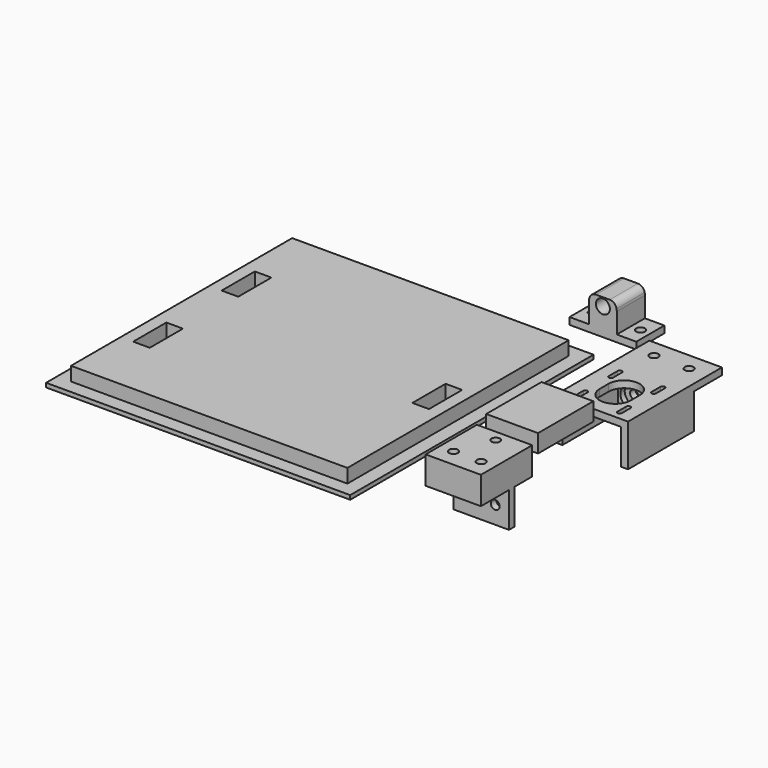
from build123d import *

# Parameters (mm, degrees)
F2_R      = 5.05
F3_DEPTH  = 25.4
F4_R      = 3.2
F5_DEPTH  = 5
F6_W      = 42.5
F6_H      = 50.5
F6_W_2    = 52.5
F6_H_2    = 25.4
F6_R      = 3.2
F7_DEPTH  = 5
F8_DEPTH  = 25.4
F9_R      = 3.2
F10_DEPTH = 9
F9_R_2    = 7.05
F11_DEPTH = 4
F12_W     = 40
F12_H     = 25.4
F12_R     = 3.2
F13_DEPTH = 15
F12_R_2   = 3.05
F14_DEPTH = 5
F15_R     = 3.2
F15_R_2   = 3.05
F16_DEPTH = 5
F17_DEPTH = 25.4
F18_R     = 3.2
F19_DEPTH = 5
F20_R     = 5.05
F20_R_2   = 3.05
F22_DEPTH = 1
F21_R     = 5.05
F21_R_2   = 3.05
F23_DEPTH = 1
F24_SIZE  = 0.99999
F26_W     = 18.7451829227
F26_H     = 8
F27_DEPTH = 25
F29_DEPTH = 8
F30_W     = 220
F30_H     = 220
F30_W_2   = 12
F30_H_2   = 30
F31_DEPTH = 3
F34_W     = 200
F34_H     = 200
F34_W_2   = 12
F34_H_2   = 30
F35_DEPTH = 10


# Not quite as in the source:
# - a fillet or chamfer is up to 0.001 mm smaller than in the source, because OpenCascade refuses the exact size
# - a feature names something its author has since deleted; it is built from what else it names


with BuildPart() as f3:
    # F2 (on offset) → F3 (new body)
    with BuildSketch(Plane.XZ.offset(-50)):
        Polygon((-65.3854490548, 5), (-79.4854490548, 5), (-79.4854490548, 0), (-31.1854490548, 0), (-31.1854490548, 5), (-45.2854490548, 5), align=None)
        with BuildLine():
            Line((-65.3854490548, 19.6345400687), (-65.3854490548, 5))
            Line((-65.3854490548, 5), (-45.2854490548, 5))
            Line((-45.2854490548, 5), (-45.2854490548, 19.6345400687))
            ThreePointArc((-45.2854490548, 19.6345400687), (-55.3354490548, 9.5845400687), (-65.3854490548, 19.6345400687))
        make_face()
        with BuildLine():
            ThreePointArc((-65.2367624625, 21.3568910211), (-65.3482084085, 20.4989185312), (-65.3854490548, 19.6345400687))
            ThreePointArc((-65.3854490548, 19.6345400687), (-55.3354490548, 9.5845400687), (-45.2854490548, 19.6345400687))
            ThreePointArc((-45.2854490548, 19.6345400687), (-45.3226897012, 20.4989185312), (-45.4341356472, 21.3568910211))
            ThreePointArc((-45.4341356472, 21.3568910211), (-47.1418128824, 24.326516373), (-50.3601622182, 25.5))
            Line((-50.3601622182, 25.5), (-60.3107358915, 25.5))
            ThreePointArc((-60.3107358915, 25.5), (-63.5290852273, 24.326516373), (-65.2367624625, 21.3568910211))
        make_face()
        with Locations((-55.3354490548, 19.6345400687)):
            Circle(F2_R, mode=Mode.SUBTRACT)
    extrude(amount=-F3_DEPTH)

    # F4 (on face) → F5 (cut, through all)
    with BuildSketch(Plane.XY.offset(5)):
        with Locations((-72.4354490548, 62.7)):
            Circle(F4_R)
        with Locations((-38.2354490548, 62.7)):
            Circle(F4_R)
    extrude(amount=-F5_DEPTH, mode=Mode.SUBTRACT)


with BuildPart() as f7:
    # F6 (on Top) → F7 (new body)
    with BuildSketch(Plane.XY):
        with Locations((0, -4)):
            Rectangle(F6_W, F6_H)
        with BuildLine():
            Line((-17.05, -23.5), (-17.05, -15.5))
            ThreePointArc((-17.05, -15.5), (-15.5, -13.95), (-13.95, -15.5))
            Line((-13.95, -15.5), (-13.95, -23.5))
            ThreePointArc((-13.95, -23.5), (-15.5, -25.05), (-17.05, -23.5))
        make_face(mode=Mode.SUBTRACT)
        with BuildLine():
            Line((-17.05, 7.5), (-17.05, 15.5))
            ThreePointArc((-17.05, 15.5), (-15.5, 17.05), (-13.95, 15.5))
            Line((-13.95, 15.5), (-13.95, 7.5))
            ThreePointArc((-13.95, 7.5), (-15.5, 5.95), (-17.05, 7.5))
        make_face(mode=Mode.SUBTRACT)
        with BuildLine():
            Line((13.95, -23.5), (13.95, -15.5))
            ThreePointArc((13.95, -15.5), (15.5, -13.95), (17.05, -15.5))
            Line((17.05, -15.5), (17.05, -23.5))
            ThreePointArc((17.05, -23.5), (15.5, -25.05), (13.95, -23.5))
        make_face(mode=Mode.SUBTRACT)
        with BuildLine():
            Line((-11.25, -8), (-11.25, 0))
            ThreePointArc((-11.25, 0), (0, 11.25), (11.25, 0))
            Line((11.25, 0), (11.25, -8))
            ThreePointArc((11.25, -8), (0, -19.25), (-11.25, -8))
        make_face(mode=Mode.SUBTRACT)
        with BuildLine():
            Line((13.95, 7.5), (13.95, 15.5))
            ThreePointArc((13.95, 15.5), (15.5, 17.05), (17.05, 15.5))
            Line((17.05, 15.5), (17.05, 7.5))
            ThreePointArc((17.05, 7.5), (15.5, 5.95), (13.95, 7.5))
        make_face(mode=Mode.SUBTRACT)
        Polygon((-21.25, 21.25), (21.25, 21.25), (21.25, -29.25), (26.25, -29.25), (26.25, 30.25), (-26.25, 30.25), (-26.25, -29.25), (-21.25, -29.25), align=None)
        with Locations((0, 42.95)):
            Rectangle(F6_W_2, F6_H_2)
        with Locations((-12.7, 42.95)):
            Circle(F6_R, mode=Mode.SUBTRACT)
        with Locations((12.7, 42.95)):
            Circle(F6_R, mode=Mode.SUBTRACT)
    extrude(amount=F7_DEPTH)

    # F6 (on Top) → F8 (join)
    with BuildSketch(Plane.XY):
        Polygon((-21.25, 21.25), (21.25, 21.25), (21.25, -29.25), (26.25, -29.25), (26.25, 30.25), (-26.25, 30.25), (-26.25, -29.25), (-21.25, -29.25), align=None)
    extrude(amount=-F8_DEPTH)

    # F9 (on face) → F10 (cut, through all)
    with BuildSketch(Plane.XZ.offset(-21.25)):
        with Locations((-12.7, -12.7)):
            Circle(F9_R)
        with Locations((12.7, -12.7)):
            Circle(F9_R)
    extrude(amount=-F10_DEPTH, mode=Mode.SUBTRACT)

    # F9 (on face) → F11 (cut)
    with BuildSketch(Plane.XZ.offset(-21.25)):
        with Locations((-12.7, -12.7)):
            Circle(F9_R_2)
        with Locations((-12.7, -12.7)):
            Circle(F9_R, mode=Mode.SUBTRACT)
        with Locations((12.7, -12.7)):
            Circle(F9_R_2)
        with Locations((12.7, -12.7)):
            Circle(F9_R, mode=Mode.SUBTRACT)
    extrude(amount=-F11_DEPTH, mode=Mode.SUBTRACT)


with BuildPart() as f13:
    # F12 (on Top) → F13 (new body)
    with BuildSketch(Plane.XY):
        Polygon((-3.313708499, -124.0808303208), (-20, -124.0808303208), (-20, -129.0808303208), (20, -129.0808303208), (20, -124.0808303208), (3.313708499, -124.0808303208), align=None)
        with Locations((0, -141.7808303208)):
            Rectangle(F12_W, F12_H)
        with Locations((-10, -141.7808303208)):
            Circle(F12_R, mode=Mode.SUBTRACT)
        with Locations((10, -141.7808303208)):
            Circle(F12_R, mode=Mode.SUBTRACT)
        Polygon((-20, -108.0808303208), (-20, -124.0808303208), (-3.313708499, -124.0808303208), (-19.313708499, -108.0808303208), align=None)
        Polygon((19.313708499, -108.0808303208), (3.313708499, -124.0808303208), (20, -124.0808303208), (20, -108.0808303208), align=None)
    extrude(amount=F13_DEPTH)

    # F12 (on Top) → F14 (join)
    with BuildSketch(Plane.XY):
        Polygon((-19.313708499, -108.0808303208), (-3.313708499, -124.0808303208), (3.313708499, -124.0808303208), (19.313708499, -108.0808303208), align=None)
        Polygon((0, -110.3073276289), (5, -113.1940789749), (5, -118.9675816668), (0, -121.8543330127), (-5, -118.9675816668), (-5, -113.1940789749), align=None, mode=Mode.SUBTRACT)
        Polygon((5, -118.9675816668), (5, -113.1940789749), (0, -110.3073276289), (-5, -113.1940789749), (-5, -118.9675816668), (0, -121.8543330127), align=None)
        with Locations((0, -116.0808303208)):
            Circle(F12_R_2, mode=Mode.SUBTRACT)
    extrude(amount=F14_DEPTH)

    # F15 (on face) → F16 (join)
    with BuildSketch(Plane.XY.offset(15)):
        Polygon((-20, -108.0808303208), (-20, -154.4808303208), (20, -154.4808303208), (20, -108.0808303208), (19.313708499, -108.0808303208), (3.313708499, -124.0808303208), (-3.313708499, -124.0808303208), (-19.313708499, -108.0808303208), align=None)
        with Locations((-10, -141.7808303208)):
            Circle(F15_R, mode=Mode.SUBTRACT)
        with Locations((10, -141.7808303208)):
            Circle(F15_R, mode=Mode.SUBTRACT)
        Polygon((19.313708499, -108.0808303208), (-19.313708499, -108.0808303208), (-3.313708499, -124.0808303208), (3.313708499, -124.0808303208), align=None)
        with Locations((0, -116.0808303208)):
            Circle(F15_R_2, mode=Mode.SUBTRACT)
    extrude(amount=F16_DEPTH)

    # F12 (on Top) → F17 (join)
    with BuildSketch(Plane.XY):
        Polygon((-3.313708499, -124.0808303208), (-20, -124.0808303208), (-20, -129.0808303208), (20, -129.0808303208), (20, -124.0808303208), (3.313708499, -124.0808303208), align=None)
    extrude(amount=-F17_DEPTH)

    # F18 (on face) → F19 (cut, through all)
    with BuildSketch(Plane.XZ.offset(129.0808303208)):
        with Locations((-10, -12.7)):
            Circle(F18_R)
        with Locations((10, -12.7)):
            Circle(F18_R)
    extrude(amount=-F19_DEPTH, mode=Mode.SUBTRACT)

    # F20 (on face) → F22 (join)
    with BuildSketch(Plane.XY.offset(5)):
        with Locations((0, -116.0808303208)):
            Circle(F20_R)
        with Locations((0, -116.0808303208)):
            Circle(F20_R_2, mode=Mode.SUBTRACT)
    extrude(amount=F22_DEPTH)

    # F21 (on face) → F23 (join)
    with BuildSketch(Plane(origin=(0, 0, 15), x_dir=(1, 0, 0), z_dir=(0, 0, -1))):
        with Locations((0, 116.0808303208)):
            Circle(F21_R)
        with Locations((0, 116.0808303208)):
            Circle(F21_R_2, mode=Mode.SUBTRACT)
    extrude(amount=F23_DEPTH)

    # F24 (size 1 in the source; OpenCascade refuses exactly that, so slightly less here)
    f24_edges = [f13.edges().sort_by_distance(p)[0] for p in [
        (-5.05, -116.08083, 6),
        (-5.05, -116.08083, 14),
    ]]
    chamfer(f24_edges, length=F24_SIZE)


with BuildPart() as f27:
    # F26 (on offset) → F27 (new body, symmetric)
    with BuildSketch(Plane.XZ.offset(80)):
        Polygon((21.7632954655, 27), (-15.7451829227, 27), (-15.7451829227, 14), (3, 14), (21.7632954655, 14), align=None)
        with Locations((-6.3725914613, 10)):
            Rectangle(F26_W, F26_H)
    extrude(amount=F27_DEPTH, both=True)

    # F28 (on face) → F29 (cut, through all)
    with BuildSketch(Plane(origin=(0, 0, 6), x_dir=(1, 0, 0), z_dir=(0, 0, -1))):
        with BuildLine():
            Line((-5.6, 105), (-8, 105))
            Line((-8, 105), (-8, 86.5))
            ThreePointArc((-8, 86.5), (-2.5, 81), (3, 86.5))
            Line((3, 86.5), (3, 89.8166247904))
            ThreePointArc((3, 89.8166247904), (2.6443375673, 89.3379112365), (2.0833333333, 89.5402393912))
            ThreePointArc((2.0833333333, 89.5402393912), (0.3277241606, 91.2174120099), (-1.9789473684, 91.9752629302))
            ThreePointArc((-1.9789473684, 91.9752629302), (-4.5593740448, 93.2661563456), (-5.6, 95.957272334))
            Line((-5.6, 95.957272334), (-5.6, 105))
        make_face()
        with BuildLine():
            Line((-6.5, 86.5), (-6.5, 91.8780567232))
            ThreePointArc((-6.5, 91.8780567232), (-6.1825741858, 92.3435313913), (-5.6333333333, 92.2179913574))
            ThreePointArc((-5.6333333333, 92.2179913574), (-4.0370096871, 91.0266553559), (-2.1210526316, 90.4820094038))
            ThreePointArc((-2.1210526316, 90.4820094038), (0.1911159884, 83.5406259552), (-6.5, 86.5))
        make_face(mode=Mode.SUBTRACT)
        with BuildLine():
            ThreePointArc((3, 86.5), (-2.5, 81), (-8, 86.5))
            Line((-8, 86.5), (-8, 73.5))
            ThreePointArc((-8, 73.5), (-2.5, 79), (3, 73.5))
            Line((3, 73.5), (3, 86.5))
        make_face()
        with BuildLine():
            ThreePointArc((3, 73.5), (-2.5, 79), (-8, 73.5))
            Line((-8, 73.5), (-8, 55))
            Line((-8, 55), (-5.6, 55))
            Line((-5.6, 55), (-5.6, 64.042727666))
            ThreePointArc((-5.6, 64.042727666), (-4.5593740448, 66.7338436544), (-1.9789473684, 68.0247370698))
            ThreePointArc((-1.9789473684, 68.0247370698), (0.3277241606, 68.7825879901), (2.0833333333, 70.4597606088))
            ThreePointArc((2.0833333333, 70.4597606088), (2.6443375673, 70.6620887635), (3, 70.1833752096))
            Line((3, 70.1833752096), (3, 73.5))
        make_face()
        with BuildLine():
            Line((-6.5, 68.1219432768), (-6.5, 73.5))
            ThreePointArc((-6.5, 73.5), (0.1911159884, 76.4593740448), (-2.1210526316, 69.5179905962))
            ThreePointArc((-2.1210526316, 69.5179905962), (-4.0370096871, 68.9733446441), (-5.6333333333, 67.7820086426))
            ThreePointArc((-5.6333333333, 67.7820086426), (-6.1825741858, 67.6564686087), (-6.5, 68.1219432768))
        make_face(mode=Mode.SUBTRACT)
    extrude(amount=-F29_DEPTH, mode=Mode.SUBTRACT)


with BuildPart() as f31:
    # F30 (on Top) → F31 (new body)
    with BuildSketch(Plane.XY):
        with Locations((-152.5378906727, -84.4977283539)):
            Rectangle(F30_W, F30_H)
        with Locations((-237.5378906727, -124.4977283539)):
            Rectangle(F30_W_2, F30_H_2, mode=Mode.SUBTRACT)
        with Locations((-237.5378906727, -44.4977283539)):
            Rectangle(F30_W_2, F30_H_2, mode=Mode.SUBTRACT)
        with Locations((-67.5378906727, -84.4977283539)):
            Rectangle(F30_W_2, F30_H_2, mode=Mode.SUBTRACT)
    extrude(amount=F31_DEPTH)

    # F34 (on face) → F35 (join)
    with BuildSketch(Plane.XY.offset(3)):
        with Locations((-152.5378906727, -84.4977283539)):
            Rectangle(F34_W, F34_H)
        with Locations((-237.5378906727, -124.4977283539)):
            Rectangle(F34_W_2, F34_H_2, mode=Mode.SUBTRACT)
        with Locations((-237.5378906727, -44.4977283539)):
            Rectangle(F34_W_2, F34_H_2, mode=Mode.SUBTRACT)
        with Locations((-67.5378906727, -84.4977283539)):
            Rectangle(F34_W_2, F34_H_2, mode=Mode.SUBTRACT)
    extrude(amount=F35_DEPTH)


solid = Compound([f3.part, f7.part, f13.part, f27.part, f31.part])
